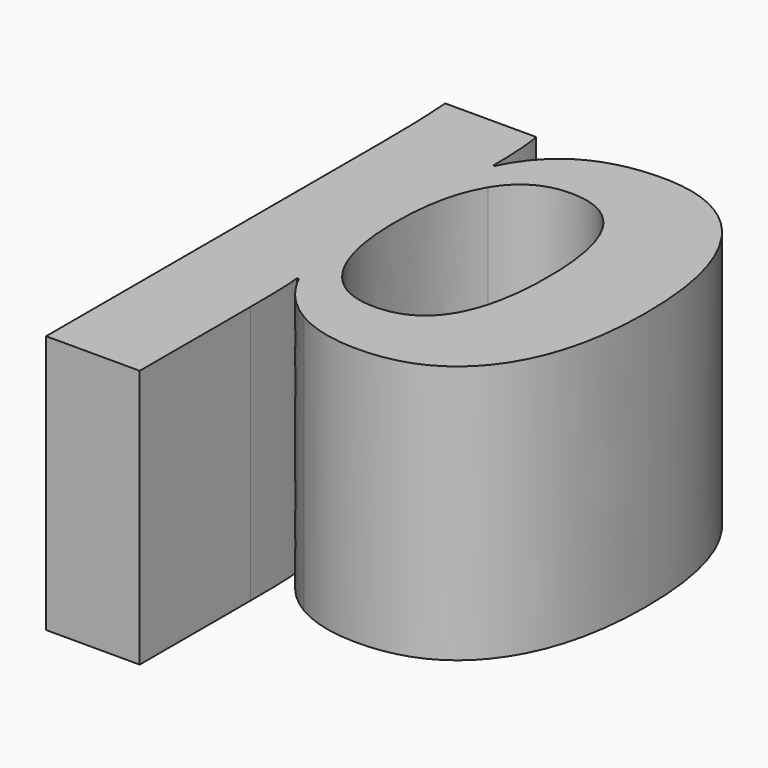
from build123d import *

# Parameters (mm, degrees)
F1_DEPTH = 25.4


with BuildPart() as f1:
    # F0 (on Top) → F1 (new body)
    with BuildSketch(Plane.XY):
        with BuildLine():
            add(Edge.make_bspline(
                [(-36.6622424432, -1.8205549519), (-36.6622424432, -10.6891040171), (-40.2117561777, -15.5160238743)],
                knots=[0, 0, 0, 1, 1, 1], degree=2))
            add(Edge.make_bspline(
                [(-40.0651685898, 11.7126205696), (-36.6622424432, 6.9537592353), (-36.6622424432, -1.8205549519)],
                knots=[0, 0, 0, 1, 1, 1], degree=2))
            add(Edge.make_bspline(
                [(-49.6561850523, 16.4714819039), (-43.4680947365, 16.4714819039), (-40.0651685898, 11.7126205696)],
                knots=[0, 0, 0, 1, 1, 1], degree=2))
            add(Edge.make_bspline(
                [(-60.974840943, 9.9588047863), (-57.8650899721, 16.4714819039), (-49.6561850523, 16.4714819039)],
                knots=[0, 0, 0, 1, 1, 1], degree=2))
            Line((-60.974840943, 9.9588047863), (-61.1004874469, 9.9588047863))
            add(Edge.make_bspline(
                [(-61.2156634088, 13.3983778299), (-61.1004874469, 11.6655031306), (-61.1004874469, 9.9588047863)],
                knots=[0, 0, 0, 1, 1, 1], degree=2))
            add(Edge.make_bspline(
                [(-61.4983680425, 15.7176028806), (-61.3308393707, 15.1312525292), (-61.2156634088, 13.3983778299)],
                knots=[0, 0, 0, 1, 1, 1], degree=2))
            Line((-61.4983680425, 15.7176028806), (-70.4297403596, 15.7176028806))
            add(Edge.make_bspline(
                [(-70.1679768099, 7.5715212127), (-70.1679768099, 12.5764402837), (-70.4297403596, 15.7176028806)],
                knots=[0, 0, 0, 1, 1, 1], degree=2))
            Line((-70.1679768099, 7.5715212127), (-70.1679768099, -33.5881793483))
            Line((-70.1679768099, -33.5881793483), (-60.974840943, -33.5881793483))
            Line((-60.974840943, -33.5881793483), (-60.974840943, -20.0078863879))
            add(Edge.make_bspline(
                [(-61.1737812408, -14.0501479958), (-60.974840943, -15.0343789428), (-60.974840943, -20.0078863879)],
                knots=[0, 0, 0, 1, 1, 1], degree=2))
            Line((-61.1737812408, -14.0501479958), (-60.974840943, -14.0501479958))
            add(Edge.make_bspline(
                [(-56.7342714373, -18.7200097231), (-59.4984945225, -17.0970757147), (-60.974840943, -14.0501479958)],
                knots=[0, 0, 0, 1, 1, 1], degree=2))
            add(Edge.make_bspline(
                [(-50.2425354037, -20.3429437315), (-53.970048352, -20.3429437315), (-56.7342714373, -18.7200097231)],
                knots=[0, 0, 0, 1, 1, 1], degree=2))
            add(Edge.make_bspline(
                [(-40.2117561777, -15.5160238743), (-43.7612699122, -20.3429437315), (-50.2425354037, -20.3429437315)],
                knots=[0, 0, 0, 1, 1, 1], degree=2))
        make_face()
        with BuildLine():
            add(Edge.make_bspline(
                [(-46.2532589057, -1.8205549519), (-46.2532589057, 10.0949218322), (-53.5512266724, 10.0949218322)],
                knots=[0, 0, 0, 1, 1, 1], degree=2))
            add(Edge.make_bspline(
                [(-53.6140499244, -14.0501479958), (-46.2532589057, -14.0501479958), (-46.2532589057, -1.8205549519)],
                knots=[0, 0, 0, 1, 1, 1], degree=2))
            add(Edge.make_bspline(
                [(-59.1582019078, -10.9299264829), (-57.2159163688, -14.0501479958), (-53.6140499244, -14.0501479958)],
                knots=[0, 0, 0, 1, 1, 1], degree=2))
            add(Edge.make_bspline(
                [(-61.1004874469, -2.0823185017), (-61.1004874469, -7.80970497), (-59.1582019078, -10.9299264829)],
                knots=[0, 0, 0, 1, 1, 1], degree=2))
            add(Edge.make_bspline(
                [(-59.1582019078, 6.8857007124), (-61.1004874469, 3.6764795926), (-61.1004874469, -2.0823185017)],
                knots=[0, 0, 0, 1, 1, 1], degree=2))
            add(Edge.make_bspline(
                [(-53.5512266724, 10.0949218322), (-57.2159163688, 10.0949218322), (-59.1582019078, 6.8857007124)],
                knots=[0, 0, 0, 1, 1, 1], degree=2))
        make_face(mode=Mode.SUBTRACT)
    extrude(amount=F1_DEPTH)


solid = f1.part
